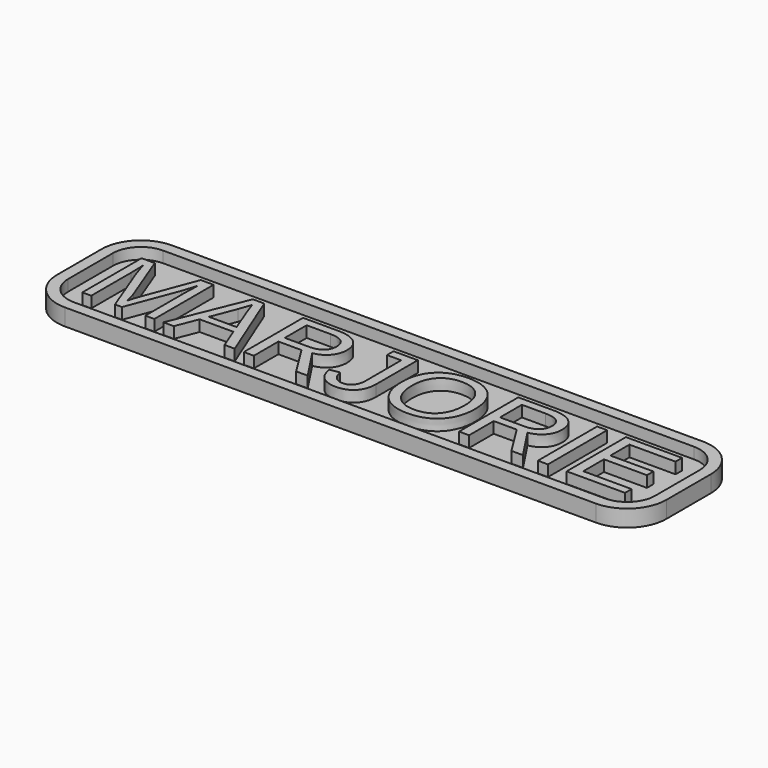
from build123d import *

# Parameters (mm, degrees)
F0_TEXT_SIZE = 19.2550694988
F1_DEPTH     = 3
F3_DEPTH     = 1


# Not quite as in the source:
# - Text() gives the source's letters only with a copy of the font that has no kerning and outlines rounded to 1/6400 em; it was checked with that copy


with BuildPart() as f1:
    # F0 (on Top) → F1 (new body)
    with BuildSketch(Plane.XY):
        with BuildLine():
            Line((54.5, 1.9318250196), (54.5, 11.9318250196))
            ThreePointArc((54.5, 11.9318250196), (52.4497474683, 16.8815724879), (47.5, 18.9318250196))
            Line((47.5, 18.9318250196), (-47.5, 18.9318250196))
            ThreePointArc((-47.5, 18.9318250196), (-52.4497474683, 16.8815724879), (-54.5, 11.9318250196))
            Line((-54.5, 11.9318250196), (-54.5, 1.9318250196))
            ThreePointArc((-54.5, 1.9318250196), (-52.4497474683, -3.0179224487), (-47.5, -5.0681749804))
            Line((-47.5, -5.0681749804), (47.5, -5.0681749804))
            ThreePointArc((47.5, -5.0681749804), (52.4497474683, -3.0179224487), (54.5, 1.9318250196))
        make_face()
        with BuildLine():
            ThreePointArc((52.5, 1.9318250196), (51.0355339059, -1.6037088864), (47.5, -3.0681749804))
            Line((47.5, -3.0681749804), (-47.5, -3.0681749804))
            ThreePointArc((-47.5, -3.0681749804), (-51.0355339059, -1.6037088864), (-52.5, 1.9318250196))
            Line((-52.5, 1.9318250196), (-52.5, 11.9318250196))
            ThreePointArc((-52.5, 11.9318250196), (-51.0355339059, 15.4673589255), (-47.5, 16.9318250196))
            Line((-47.5, 16.9318250196), (47.5, 16.9318250196))
            ThreePointArc((47.5, 16.9318250196), (51.0355339059, 15.4673589255), (52.5, 11.9318250196))
            Line((52.5, 11.9318250196), (52.5, 1.9318250196))
        make_face(mode=Mode.SUBTRACT)
        with Locations((-50, 0)):
            Text('MARJORIE', F0_TEXT_SIZE, font='Arimo', text_align=(TextAlign.LEFT, TextAlign.BOTTOM))
    extrude(amount=F1_DEPTH)

    # F2 (on Top) → F3 (join)
    with BuildSketch(Plane.XY):
        with BuildLine():
            ThreePointArc((54.5, 11.9318250196), (52.4497474683, 16.8815724879), (47.5, 18.9318250196))
            Line((47.5, 18.9318250196), (-47.5, 18.9318250196))
            ThreePointArc((-47.5, 18.9318250196), (-52.4497474683, 16.8815724879), (-54.5, 11.9318250196))
            Line((-54.5, 11.9318250196), (-54.5, 1.9318250196))
            ThreePointArc((-54.5, 1.9318250196), (-52.4497474683, -3.0179224487), (-47.5, -5.0681749804))
            Line((-47.5, -5.0681749804), (47.5, -5.0681749804))
            ThreePointArc((47.5, -5.0681749804), (52.4497474683, -3.0179224487), (54.5, 1.9318250196))
            Line((54.5, 1.9318250196), (54.5, 11.9318250196))
        make_face()
    extrude(amount=F3_DEPTH)


solid = f1.part
